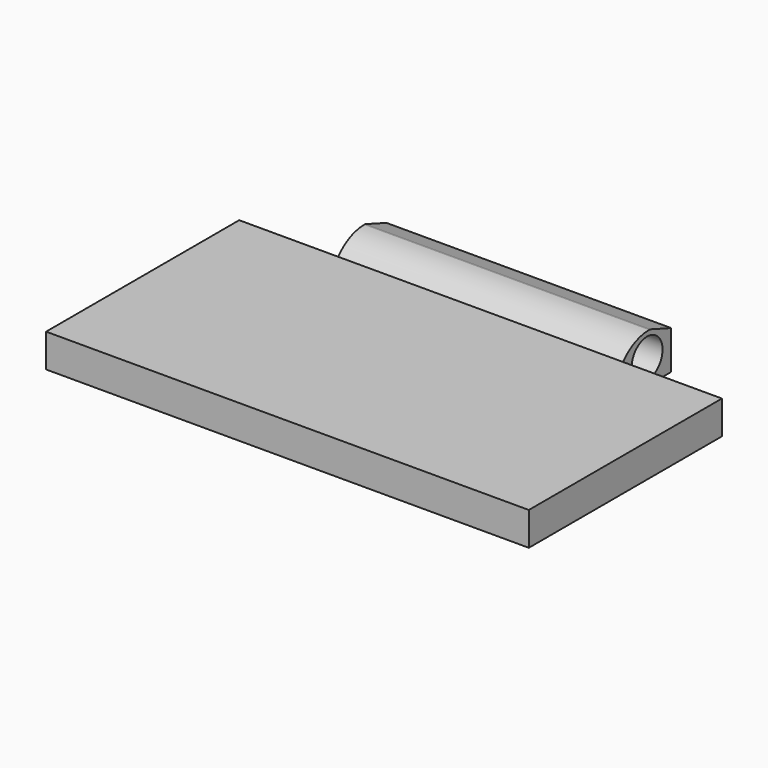
from build123d import *

# Parameters (mm, degrees)
F0_W        = 59
F0_H        = 12.5
F1_DEPTH    = 10
F2_DEPTH    = 6.9
F3_R        = 4
F4_DEPTH    = 59
F5_T1_DEPTH = 92.9816126751
F6_SIZE2    = 5.4949548389
F6_SIZE     = 2


# Not quite as in the source:
# - a fillet or chamfer that OpenCascade refuses, or shapes differently, is made with other operations: its cross-section is extruded or revolved along the edge and cut away or added


with BuildPart() as f1:
    # F0 (on Top) → F1 (new body)
    with BuildSketch(Plane.XY):
        with Locations((0, 31.25)):
            Rectangle(F0_W, F0_H)
    extrude(amount=F1_DEPTH)

    # F0 (on Top) → F2 (join)
    with BuildSketch(Plane.XY):
        Polygon((-50, -25), (50, -25), (50, 25), (29.5, 25), (-29.5, 25), (-50, 25), align=None)
    extrude(amount=F2_DEPTH)

    # F3 (on face) → F4 (cut, through all)
    with BuildSketch(Plane.YZ.offset(29.5)):
        with Locations((31.25, 5)):
            Circle(F3_R)
    extrude(amount=-F4_DEPTH, mode=Mode.SUBTRACT)

    # F5: fillet of radius 9 on 1 edges, made by hand

    # F5_s2 → F5_t1 (cut)
    with BuildSketch(Plane.YZ.offset(-46.4908063375)):
        with BuildLine():
            ThreePointArc((25, 6.9), (28.0613526556, 9.1884064384), (31.796322535, 10))
            Line((31.796322535, 10), (25, 10))
            Line((25, 10), (25, 6.9))
        make_face()
    extrude(amount=F5_T1_DEPTH, mode=Mode.SUBTRACT)

    # F6
    f6_edges = [f1.edges().sort_by_distance(p)[0] for p in [
        (0, 37.5, 10),
    ]]
    f6_side = f1.faces().sort_by_distance((0, 37.5, 5))[0]
    chamfer(f6_edges, length=F6_SIZE, length2=F6_SIZE2, reference=f6_side)


solid = f1.part
